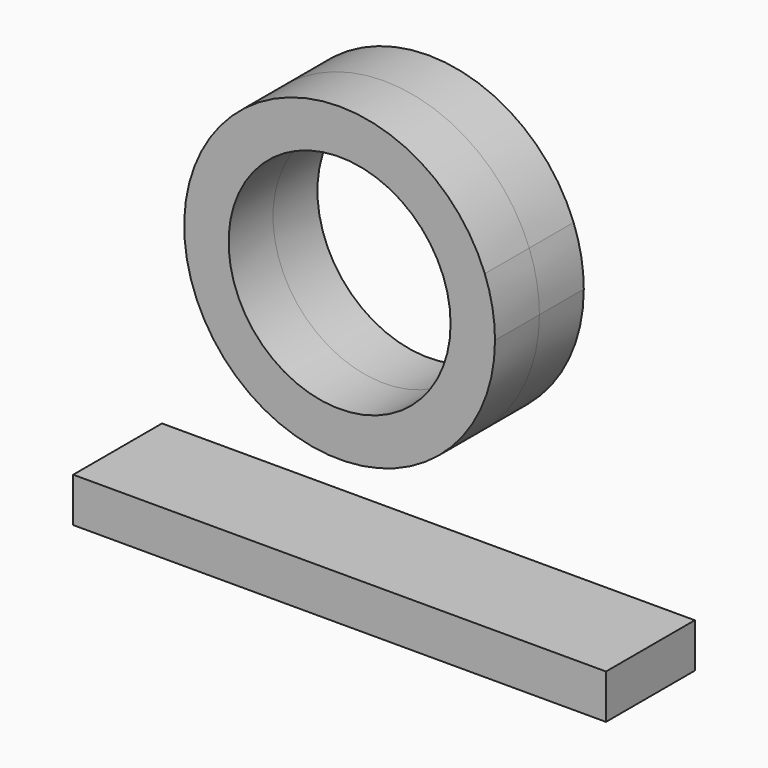
from build123d import *

# Parameters (mm, degrees)
F0_R     = 25
F1_DEPTH = 12.5
F0_W     = 120
F0_H     = 10


# Not quite as in the source:
# - a feature names something its author has since deleted; it is built from what else it names


with BuildPart() as f1:
    # F0 (on Front) → F1 (new body, symmetric)
    with BuildSketch(Plane.XZ):
        with BuildLine():
            ThreePointArc((-32.7034839498, 12.4692476737), (-6.3394819094, -34.4210832067), (35, 0))
            ThreePointArc((35, 0), (34.4210832067, 6.3394819094), (32.7034839498, 12.4692476737))
            ThreePointArc((32.7034839498, 12.4692476737), (0, 35), (-32.7034839498, 12.4692476737))
        make_face()
        Circle(F0_R, mode=Mode.SUBTRACT)
    extrude(amount=F1_DEPTH, both=True)


with BuildPart() as f1b:
    # F0 (on Front) → F1, piece 2 (new body, symmetric)
    with BuildSketch(Plane.XZ):
        with Locations((0, -62.5307523263)):
            Rectangle(F0_W, F0_H)
    extrude(amount=F1_DEPTH, both=True)


solid = Compound([f1.part, f1b.part])
